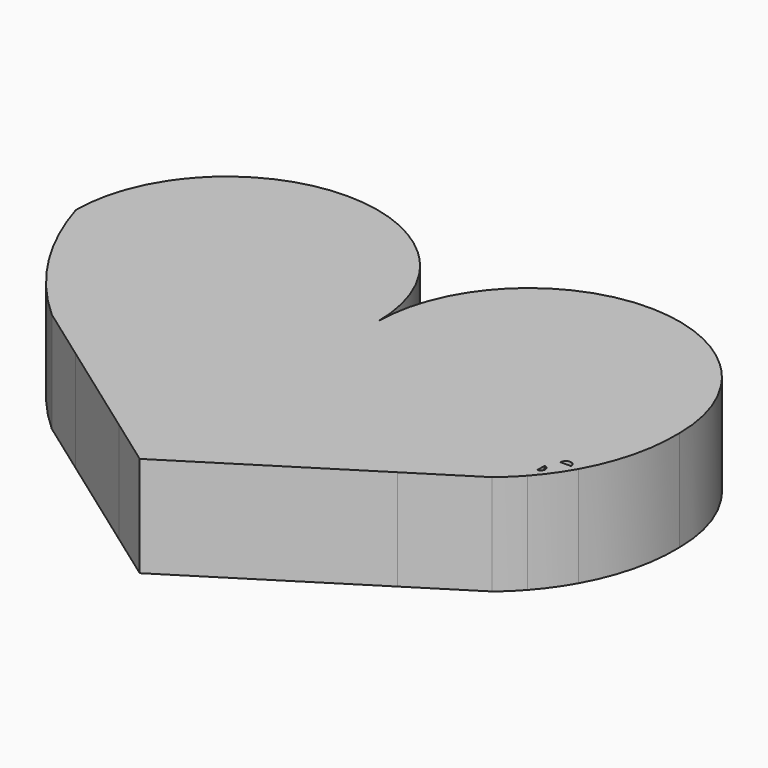
from build123d import *

# Parameters (mm, degrees)
F1_DEPTH = 25.4


with BuildPart() as f1:
    # F0 (on Top) → F1 (new body)
    with BuildSketch(Plane.XY):
        with BuildLine():
            Line((7.3731103912, 0), (0, 0))
            Line((0, 0), (-3.0946007464, 0))
            ThreePointArc((-3.0946007464, 0), (2.1392548224, -6.2743292812), (7.3731103912, 0))
        make_face()
        with BuildLine():
            ThreePointArc((69.9874537027, 20.8518655366), (67.2803767578, 24.4972572398), (64.1588523404, 27.7947155895))
            Line((64.1588523404, 27.7947155895), (64.1588523404, 25.8992332965))
            Line((64.1588523404, 25.8992332965), (64.1588523404, 20.8518655366))
            Line((64.1588523404, 20.8518655366), (65.8508837223, 20.8518655366))
            Line((65.8508837223, 20.8518655366), (68.7087923288, 20.8518655366))
            Line((68.7087923288, 20.8518655366), (69.9874537027, 20.8518655366))
        make_face()
        with BuildLine():
            ThreePointArc((13.9820705187, 29.494668629), (9.7658289741, 25.4712534493), (6.2125462973, 20.8518655366))
            Line((6.2125462973, 20.8518655366), (7.9780612141, 20.8518655366))
            ThreePointArc((7.9780612141, 20.8518655366), (10.7168983668, 23.5907026893), (13.4557355195, 20.8518655366))
            Line((13.4557355195, 20.8518655366), (13.9820705187, 20.8518655366))
            Line((13.9820705187, 20.8518655366), (13.9820705187, 23.8748770207))
            ThreePointArc((13.9820705187, 23.8748770207), (11.8386334758, 26.0183140635), (13.9820705187, 28.1617511064))
            Line((13.9820705187, 28.1617511064), (13.9820705187, 29.494668629))
        make_face()
        with BuildLine():
            Line((-8.6229192093, 20.8518655366), (-6.2125462973, 20.8518655366))
            ThreePointArc((-6.2125462973, 20.8518655366), (-9.0177469774, 24.613666105), (-12.2641128277, 28.0020880296))
            Line((-12.2641128277, 28.0020880296), (-12.2641128277, 25.3109112382))
            Line((-12.2641128277, 25.3109112382), (-12.2641128277, 22.7124486119))
            Line((-12.2641128277, 22.7124486119), (-12.2641128277, 20.8518655366))
            Line((-12.2641128277, 20.8518655366), (-10.6853200123, 20.8518655366))
            Line((-10.6853200123, 20.8518655366), (-8.6229192093, 20.8518655366))
        make_face()
        with BuildLine():
            Line((-64.0826212534, 25.3109112382), (-64.0826212534, 27.8659898945))
            ThreePointArc((-64.0826212534, 27.8659898945), (-67.2467987777, 24.5371987198), (-69.9874537027, 20.8518655366))
            Line((-69.9874537027, 20.8518655366), (-68.3164224029, 20.8518655366))
            ThreePointArc((-68.3164224029, 20.8518655366), (-66.9433735311, 22.1881347575), (-65.5703246593, 20.8518655366))
            Line((-65.5703246593, 20.8518655366), (-64.0826212534, 20.8518655366))
            Line((-64.0826212534, 20.8518655366), (-64.0826212534, 22.7124486119))
            ThreePointArc((-64.0826212534, 22.7124486119), (-65.3282893316, 24.011679925), (-64.0826212534, 25.3109112382))
        make_face()
        with BuildLine():
            Line((-72.4636018276, 0), (-76.2, 0))
            ThreePointArc((-76.2, 0), (-71.1383173271, -12.6890619161), (-64.0826212534, -24.3873556682))
            Line((-64.0826212534, -24.3873556682), (-64.0826212534, -17.1742849052))
            ThreePointArc((-64.0826212534, -17.1742849052), (-67.6059327944, -12.0701026171), (-64.0826212534, -6.9659203291))
            Line((-64.0826212534, -6.9659203291), (-64.0826212534, 0))
            Line((-64.0826212534, 0), (-66.7451322079, 0))
            ThreePointArc((-66.7451322079, 0), (-69.6043670177, -2.4147276963), (-72.4636018276, 0))
        make_face()
        with BuildLine():
            Line((-56.3778951764, -24.3873556682), (-64.0826212534, -24.3873556682))
            ThreePointArc((-64.0826212534, -24.3873556682), (-58.4160274717, -31.4204459437), (-52.0255934776, -37.8030000781))
            Line((-52.0255934776, -37.8030000781), (-38.1, -47.7827715515))
            Line((-38.1, -47.7827715515), (-38.1, -40.8103056252))
            ThreePointArc((-38.1, -40.8103056252), (-43.5800189721, -35.9057448804), (-38.1, -31.0011841357))
            Line((-38.1, -31.0011841357), (-38.1, -24.3873556682))
            Line((-38.1, -24.3873556682), (-45.1089218259, -24.3873556682))
            Line((-45.1089218259, -24.3873556682), (-56.3778951764, -24.3873556682))
        make_face()
        with BuildLine():
            ThreePointArc((64.1588523404, -32.9412611677), (67.4447841374, -28.8340923774), (70.2541819173, -24.3873556682))
            Line((70.2541819173, -24.3873556682), (68.3325305581, -24.3873556682))
            Line((68.3325305581, -24.3873556682), (65.6523033977, -24.3873556682))
            Line((65.6523033977, -24.3873556682), (64.1588523404, -24.3873556682))
            Line((64.1588523404, -24.3873556682), (64.1588523404, -27.585182339))
            ThreePointArc((64.1588523404, -27.585182339), (65.2624770419, -28.6888070405), (64.1588523404, -29.792431742))
            Line((64.1588523404, -29.792431742), (64.1588523404, -32.9412611677))
        make_face()
        with BuildLine():
            Line((-12.2641128277, -52.9070980847), (-12.2641128277, -47.7827715515))
            Line((-12.2641128277, -47.7827715515), (-18.7669228762, -47.7827715515))
            Line((-18.7669228762, -47.7827715515), (-29.9223959446, -47.7827715515))
            Line((-29.9223959446, -47.7827715515), (-38.1, -47.7827715515))
            Line((-38.1, -47.7827715515), (-12.2641128277, -66.2980506459))
            Line((-12.2641128277, -66.2980506459), (-12.2641128277, -61.5275651217))
            ThreePointArc((-12.2641128277, -61.5275651217), (-16.9211194514, -57.2173316032), (-12.2641128277, -52.9070980847))
        make_face()
        Polygon((21.1353525519, -47.7827715515), (13.9820705187, -47.7827715515), (13.9820705187, -54.9595914781), (13.9820705187, -60.7065707445), (13.9820705187, -66.2672672047), (43.2854445061, -47.7827715515), (35.3846773505, -47.7827715515), align=None)
        with BuildLine():
            ThreePointArc((76.2, 0), (74.6138465933, 10.878832978), (69.9874537027, 20.8518655366))
            Line((69.9874537027, 20.8518655366), (68.7087923288, 20.8518655366))
            ThreePointArc((68.7087923288, 20.8518655366), (67.2798380256, 19.4229112333), (65.8508837223, 20.8518655366))
            Line((65.8508837223, 20.8518655366), (64.1588523404, 20.8518655366))
            Line((64.1588523404, 20.8518655366), (64.1588523404, 15.7774444669))
            Line((64.1588523404, 15.7774444669), (64.1588523404, 4.3457765132))
            Line((64.1588523404, 4.3457765132), (64.1588523404, 0))
            Line((64.1588523404, 0), (76.2, 0))
        make_face()
        with BuildLine():
            ThreePointArc((70.2541819173, -24.3873556682), (74.8750675455, -12.5954667415), (76.2, 0))
            Line((76.2, 0), (64.1588523404, 0))
            Line((64.1588523404, 0), (64.1588523404, -7.877567783))
            ThreePointArc((64.1588523404, -7.877567783), (69.0336172821, -12.7523327246), (64.1588523404, -17.6270976663))
            Line((64.1588523404, -17.6270976663), (64.1588523404, -24.3873556682))
            Line((64.1588523404, -24.3873556682), (65.6523033977, -24.3873556682))
            ThreePointArc((65.6523033977, -24.3873556682), (66.9924169779, -23.0472420879), (68.3325305581, -24.3873556682))
            Line((68.3325305581, -24.3873556682), (70.2541819173, -24.3873556682))
        make_face()
        with BuildLine():
            ThreePointArc((64.1588523404, 27.7947155895), (54.4953024728, 34.3919184813), (43.2854445061, 37.7454787395))
            Line((43.2854445061, 37.7454787395), (43.2854445061, 33.5203446448))
            Line((43.2854445061, 33.5203446448), (43.2854445061, 24.9465927482))
            Line((43.2854445061, 24.9465927482), (43.2854445061, 20.8518655366))
            Line((43.2854445061, 20.8518655366), (48.5843010247, 20.8518655366))
            Line((48.5843010247, 20.8518655366), (60.2541230619, 20.8518655366))
            Line((60.2541230619, 20.8518655366), (63.1740450807, 20.8518655366))
            ThreePointArc((63.1740450807, 20.8518655366), (61.5875799588, 23.7811638152), (64.1588523404, 25.8992332965))
            Line((64.1588523404, 25.8992332965), (64.1588523404, 27.7947155895))
        make_face()
        with BuildLine():
            ThreePointArc((43.2854445061, 37.7454787395), (27.7738819635, 36.6739865067), (13.9820705187, 29.494668629))
            Line((13.9820705187, 29.494668629), (13.9820705187, 28.1617511064))
            Line((13.9820705187, 28.1617511064), (13.9820705187, 23.8748770207))
            Line((13.9820705187, 23.8748770207), (13.9820705187, 20.8518655366))
            Line((13.9820705187, 20.8518655366), (22.616366089, 20.8518655366))
            ThreePointArc((22.616366089, 20.8518655366), (28.9394616748, 27.1749611223), (35.2625572606, 20.8518655366))
            Line((35.2625572606, 20.8518655366), (43.2854445061, 20.8518655366))
            Line((43.2854445061, 20.8518655366), (43.2854445061, 24.9465927482))
            ThreePointArc((43.2854445061, 24.9465927482), (38.9985685578, 29.2334686965), (43.2854445061, 33.5203446448))
            Line((43.2854445061, 33.5203446448), (43.2854445061, 37.7454787395))
        make_face()
        with BuildLine():
            ThreePointArc((6.2125462973, 20.8518655366), (1.5861534067, 10.878832978), (0, 0))
            Line((0, 0), (7.3731103912, 0))
            Line((7.3731103912, 0), (13.9820705187, 0))
            Line((13.9820705187, 0), (13.9820705187, 4.531538114))
            Line((13.9820705187, 4.531538114), (13.9820705187, 13.5946199298))
            Line((13.9820705187, 13.5946199298), (13.9820705187, 20.8518655366))
            Line((13.9820705187, 20.8518655366), (13.4557355195, 20.8518655366))
            Line((13.4557355195, 20.8518655366), (7.9780612141, 20.8518655366))
            Line((7.9780612141, 20.8518655366), (6.2125462973, 20.8518655366))
        make_face()
        with BuildLine():
            Line((-3.0946007464, 0), (0, 0))
            ThreePointArc((0, 0), (-1.5861534067, 10.878832978), (-6.2125462973, 20.8518655366))
            Line((-6.2125462973, 20.8518655366), (-8.6229192093, 20.8518655366))
            ThreePointArc((-8.6229192093, 20.8518655366), (-9.6541196108, 18.7953565289), (-10.6853200123, 20.8518655366))
            Line((-10.6853200123, 20.8518655366), (-12.2641128277, 20.8518655366))
            Line((-12.2641128277, 20.8518655366), (-12.2641128277, 13.5718295351))
            ThreePointArc((-12.2641128277, 13.5718295351), (-6.9563915031, 10.103298584), (-12.2641128277, 6.6347676329))
            Line((-12.2641128277, 6.6347676329), (-12.2641128277, 0))
            Line((-12.2641128277, 0), (-3.0946007464, 0))
        make_face()
        with BuildLine():
            Line((-12.2641128277, 25.3109112382), (-12.2641128277, 28.0020880296))
            ThreePointArc((-12.2641128277, 28.0020880296), (-24.2304209496, 35.4858391047), (-38.1, 38.1))
            Line((-38.1, 38.1), (-38.1, 33.7021276355))
            Line((-38.1, 33.7021276355), (-38.1, 25.3109112382))
            Line((-38.1, 25.3109112382), (-38.1, 20.8518655366))
            Line((-38.1, 20.8518655366), (-32.246787101, 20.8518655366))
            Line((-32.246787101, 20.8518655366), (-17.6224876195, 20.8518655366))
            Line((-17.6224876195, 20.8518655366), (-12.2641128277, 20.8518655366))
            Line((-12.2641128277, 20.8518655366), (-12.2641128277, 22.7124486119))
            ThreePointArc((-12.2641128277, 22.7124486119), (-15.2984271998, 24.011679925), (-12.2641128277, 25.3109112382))
        make_face()
        with BuildLine():
            Line((-38.1, 33.7021276355), (-38.1, 38.1))
            ThreePointArc((-38.1, 38.1), (-52.0627322724, 35.4492892382), (-64.0826212534, 27.8659898945))
            Line((-64.0826212534, 27.8659898945), (-64.0826212534, 25.3109112382))
            Line((-64.0826212534, 25.3109112382), (-64.0826212534, 22.7124486119))
            Line((-64.0826212534, 22.7124486119), (-64.0826212534, 20.8518655366))
            Line((-64.0826212534, 20.8518655366), (-55.4025620222, 20.8518655366))
            ThreePointArc((-55.4025620222, 20.8518655366), (-49.9948691577, 25.7247809767), (-44.5871762931, 20.8518655366))
            Line((-44.5871762931, 20.8518655366), (-38.1, 20.8518655366))
            Line((-38.1, 20.8518655366), (-38.1, 25.3109112382))
            ThreePointArc((-38.1, 25.3109112382), (-43.0000966156, 29.5065194368), (-38.1, 33.7021276355))
        make_face()
        with BuildLine():
            Line((-68.3164224029, 20.8518655366), (-69.9874537027, 20.8518655366))
            ThreePointArc((-69.9874537027, 20.8518655366), (-74.6138465933, 10.878832978), (-76.2, 0))
            Line((-76.2, 0), (-72.4636018276, 0))
            Line((-72.4636018276, 0), (-66.7451322079, 0))
            Line((-66.7451322079, 0), (-64.0826212534, 0))
            Line((-64.0826212534, 0), (-64.0826212534, 5.2506080829))
            ThreePointArc((-64.0826212534, 5.2506080829), (-68.2045203392, 9.7503920551), (-64.0826212534, 14.2501760274))
            Line((-64.0826212534, 14.2501760274), (-64.0826212534, 20.8518655366))
            Line((-64.0826212534, 20.8518655366), (-65.5703246593, 20.8518655366))
            Line((-65.5703246593, 20.8518655366), (-68.3164224029, 20.8518655366))
        make_face()
        with BuildLine():
            Line((48.8840192556, -24.3873556682), (43.2854445061, -24.3873556682))
            Line((43.2854445061, -24.3873556682), (43.2854445061, -29.2515400797))
            Line((43.2854445061, -29.2515400797), (43.2854445061, -44.1332776099))
            Line((43.2854445061, -44.1332776099), (43.2854445061, -47.7827715515))
            Line((43.2854445061, -47.7827715515), (59.106323868, -37.8030000781))
            ThreePointArc((59.106323868, -37.8030000781), (61.7228361509, -35.46592028), (64.1588523404, -32.9412611677))
            Line((64.1588523404, -32.9412611677), (64.1588523404, -29.792431742))
            Line((64.1588523404, -29.792431742), (64.1588523404, -27.585182339))
            Line((64.1588523404, -27.585182339), (64.1588523404, -24.3873556682))
            Line((64.1588523404, -24.3873556682), (63.8832971454, -24.3873556682))
            ThreePointArc((63.8832971454, -24.3873556682), (56.3836582005, -31.886994613), (48.8840192556, -24.3873556682))
        make_face()
        with BuildLine():
            Line((13.9820705187, -54.9595914781), (13.9820705187, -47.7827715515))
            Line((13.9820705187, -47.7827715515), (5.5258679204, -47.7827715515))
            ThreePointArc((5.5258679204, -47.7827715515), (-0.3237351775, -55.877302251), (-6.1733382754, -47.7827715515))
            Line((-6.1733382754, -47.7827715515), (-12.2641128277, -47.7827715515))
            Line((-12.2641128277, -47.7827715515), (-12.2641128277, -52.9070980847))
            Line((-12.2641128277, -52.9070980847), (-12.2641128277, -61.5275651217))
            Line((-12.2641128277, -61.5275651217), (-12.2641128277, -66.2980506459))
            Line((-12.2641128277, -66.2980506459), (0, -75.0871226192))
            Line((0, -75.0871226192), (13.9820705187, -66.2672672047))
            Line((13.9820705187, -66.2672672047), (13.9820705187, -60.7065707445))
            ThreePointArc((13.9820705187, -60.7065707445), (8.35846738, -57.8330811113), (13.9820705187, -54.9595914781))
        make_face()
        with BuildLine():
            Line((-38.1, -6.2933946028), (-38.1, 0))
            Line((-38.1, 0), (-46.1211204529, 0))
            Line((-46.1211204529, 0), (-55.3081780672, 0))
            Line((-55.3081780672, 0), (-64.0826212534, 0))
            Line((-64.0826212534, 0), (-64.0826212534, -6.9659203291))
            Line((-64.0826212534, -6.9659203291), (-64.0826212534, -17.1742849052))
            Line((-64.0826212534, -17.1742849052), (-64.0826212534, -24.3873556682))
            Line((-64.0826212534, -24.3873556682), (-56.3778951764, -24.3873556682))
            ThreePointArc((-56.3778951764, -24.3873556682), (-50.7434085011, -16.8907498785), (-45.1089218259, -24.3873556682))
            Line((-45.1089218259, -24.3873556682), (-38.1, -24.3873556682))
            Line((-38.1, -24.3873556682), (-38.1, -20.0098585337))
            Line((-38.1, -20.0098585337), (-38.1, -6.2933946028))
        make_face()
        with BuildLine():
            Line((-12.2641128277, -32.1551971138), (-12.2641128277, -24.3873556682))
            Line((-12.2641128277, -24.3873556682), (-20.3056093305, -24.3873556682))
            ThreePointArc((-20.3056093305, -24.3873556682), (-24.0561561659, -29.287069319), (-27.8067030013, -24.3873556682))
            Line((-27.8067030013, -24.3873556682), (-38.1, -24.3873556682))
            Line((-38.1, -24.3873556682), (-38.1, -31.0011841357))
            Line((-38.1, -31.0011841357), (-38.1, -40.8103056252))
            Line((-38.1, -40.8103056252), (-38.1, -47.7827715515))
            Line((-38.1, -47.7827715515), (-29.9223959446, -47.7827715515))
            ThreePointArc((-29.9223959446, -47.7827715515), (-24.3446594104, -38.7493341849), (-18.7669228762, -47.7827715515))
            Line((-18.7669228762, -47.7827715515), (-12.2641128277, -47.7827715515))
            Line((-12.2641128277, -47.7827715515), (-12.2641128277, -41.0026423633))
            Line((-12.2641128277, -41.0026423633), (-12.2641128277, -32.1551971138))
        make_face()
        with BuildLine():
            Line((21.5103328228, -24.3873556682), (13.9820705187, -24.3873556682))
            Line((13.9820705187, -24.3873556682), (13.9820705187, -31.7664258182))
            Line((13.9820705187, -31.7664258182), (13.9820705187, -41.6183918715))
            Line((13.9820705187, -41.6183918715), (13.9820705187, -47.7827715515))
            Line((13.9820705187, -47.7827715515), (21.1353525519, -47.7827715515))
            ThreePointArc((21.1353525519, -47.7827715515), (28.2600149512, -40.6581091522), (35.3846773505, -47.7827715515))
            Line((35.3846773505, -47.7827715515), (43.2854445061, -47.7827715515))
            Line((43.2854445061, -47.7827715515), (43.2854445061, -44.1332776099))
            ThreePointArc((43.2854445061, -44.1332776099), (35.844575741, -36.6924088448), (43.2854445061, -29.2515400797))
            Line((43.2854445061, -29.2515400797), (43.2854445061, -24.3873556682))
            Line((43.2854445061, -24.3873556682), (35.7596613467, -24.3873556682))
            Line((35.7596613467, -24.3873556682), (21.5103328228, -24.3873556682))
        make_face()
        with BuildLine():
            Line((13.9820705187, 0), (7.3731103912, 0))
            ThreePointArc((7.3731103912, 0), (2.1392548224, -6.2743292812), (-3.0946007464, 0))
            Line((-3.0946007464, 0), (-12.2641128277, 0))
            Line((-12.2641128277, 0), (-12.2641128277, -8.9736226946))
            ThreePointArc((-12.2641128277, -8.9736226946), (-8.4361824744, -13.0727961659), (-12.2641128277, -17.1719696373))
            Line((-12.2641128277, -17.1719696373), (-12.2641128277, -24.3873556682))
            Line((-12.2641128277, -24.3873556682), (-7.1995845065, -24.3873556682))
            Line((-7.1995845065, -24.3873556682), (6.9626118056, -24.3873556682))
            Line((6.9626118056, -24.3873556682), (13.9820705187, -24.3873556682))
            Line((13.9820705187, -24.3873556682), (13.9820705187, -18.3862992879))
            Line((13.9820705187, -18.3862992879), (13.9820705187, -9.394259192))
            Line((13.9820705187, -9.394259192), (13.9820705187, 0))
        make_face()
        with BuildLine():
            Line((-12.2641128277, -8.9736226946), (-12.2641128277, 0))
            Line((-12.2641128277, 0), (-19.0984625369, 0))
            ThreePointArc((-19.0984625369, 0), (-24.9319020659, -6.3078507166), (-30.7653415948, 0))
            Line((-30.7653415948, 0), (-38.1, 0))
            Line((-38.1, 0), (-38.1, -6.2933946028))
            ThreePointArc((-38.1, -6.2933946028), (-32.493432726, -13.1516265683), (-38.1, -20.0098585337))
            Line((-38.1, -20.0098585337), (-38.1, -24.3873556682))
            Line((-38.1, -24.3873556682), (-27.8067030013, -24.3873556682))
            Line((-27.8067030013, -24.3873556682), (-20.3056093305, -24.3873556682))
            Line((-20.3056093305, -24.3873556682), (-12.2641128277, -24.3873556682))
            Line((-12.2641128277, -24.3873556682), (-12.2641128277, -17.1719696373))
            Line((-12.2641128277, -17.1719696373), (-12.2641128277, -8.9736226946))
        make_face()
        with BuildLine():
            Line((20.543390885, 0), (13.9820705187, 0))
            Line((13.9820705187, 0), (13.9820705187, -9.394259192))
            ThreePointArc((13.9820705187, -9.394259192), (20.7282060591, -13.89027924), (13.9820705187, -18.3862992879))
            Line((13.9820705187, -18.3862992879), (13.9820705187, -24.3873556682))
            Line((13.9820705187, -24.3873556682), (21.5103328228, -24.3873556682))
            ThreePointArc((21.5103328228, -24.3873556682), (28.6349970847, -17.2626914062), (35.7596613467, -24.3873556682))
            Line((35.7596613467, -24.3873556682), (43.2854445061, -24.3873556682))
            Line((43.2854445061, -24.3873556682), (43.2854445061, -21.2359833103))
            ThreePointArc((43.2854445061, -21.2359833103), (35.176776054, -13.1273148581), (43.2854445061, -5.018646406))
            Line((43.2854445061, -5.018646406), (43.2854445061, 0))
            Line((43.2854445061, 0), (31.3057955354, 0))
            Line((31.3057955354, 0), (20.543390885, 0))
        make_face()
        Polygon((47.1553392708, 0), (43.2854445061, 0), (43.2854445061, -5.018646406), (43.2854445061, -21.2359833103), (43.2854445061, -24.3873556682), (48.8840192556, -24.3873556682), (63.8832971454, -24.3873556682), (64.1588523404, -24.3873556682), (64.1588523404, -17.6270976663), (64.1588523404, -7.877567783), (64.1588523404, 0), (60.4922883213, 0), align=None)
        with BuildLine():
            Line((13.9820705187, 4.531538114), (13.9820705187, 0))
            Line((13.9820705187, 0), (20.543390885, 0))
            ThreePointArc((20.543390885, 0), (25.9245932102, 5.3812023252), (31.3057955354, 0))
            Line((31.3057955354, 0), (43.2854445061, 0))
            Line((43.2854445061, 0), (43.2854445061, 9.0630790219))
            ThreePointArc((43.2854445061, 9.0630790219), (38.119115994, 14.229407534), (43.2854445061, 19.3957360461))
            Line((43.2854445061, 19.3957360461), (43.2854445061, 20.8518655366))
            Line((43.2854445061, 20.8518655366), (35.2625572606, 20.8518655366))
            Line((35.2625572606, 20.8518655366), (22.616366089, 20.8518655366))
            Line((22.616366089, 20.8518655366), (13.9820705187, 20.8518655366))
            Line((13.9820705187, 20.8518655366), (13.9820705187, 13.5946199298))
            ThreePointArc((13.9820705187, 13.5946199298), (18.5136114266, 9.0630790219), (13.9820705187, 4.531538114))
        make_face()
        with BuildLine():
            Line((43.2854445061, 9.0630790219), (43.2854445061, 0))
            Line((43.2854445061, 0), (47.1553392708, 0))
            ThreePointArc((47.1553392708, 0), (53.823813796, 6.6684745252), (60.4922883213, 0))
            Line((60.4922883213, 0), (64.1588523404, 0))
            Line((64.1588523404, 0), (64.1588523404, 4.3457765132))
            ThreePointArc((64.1588523404, 4.3457765132), (58.4430183636, 10.0616104901), (64.1588523404, 15.7774444669))
            Line((64.1588523404, 15.7774444669), (64.1588523404, 20.8518655366))
            Line((64.1588523404, 20.8518655366), (63.1740450807, 20.8518655366))
            Line((63.1740450807, 20.8518655366), (60.2541230619, 20.8518655366))
            ThreePointArc((60.2541230619, 20.8518655366), (54.4192120433, 15.016954518), (48.5843010247, 20.8518655366))
            Line((48.5843010247, 20.8518655366), (43.2854445061, 20.8518655366))
            Line((43.2854445061, 20.8518655366), (43.2854445061, 19.3957360461))
            Line((43.2854445061, 19.3957360461), (43.2854445061, 9.0630790219))
        make_face()
        with BuildLine():
            Line((-19.0984625369, 0), (-12.2641128277, 0))
            Line((-12.2641128277, 0), (-12.2641128277, 6.6347676329))
            Line((-12.2641128277, 6.6347676329), (-12.2641128277, 13.5718295351))
            Line((-12.2641128277, 13.5718295351), (-12.2641128277, 20.8518655366))
            Line((-12.2641128277, 20.8518655366), (-17.6224876195, 20.8518655366))
            ThreePointArc((-17.6224876195, 20.8518655366), (-24.9346373603, 15.1396827417), (-32.246787101, 20.8518655366))
            Line((-32.246787101, 20.8518655366), (-38.1, 20.8518655366))
            Line((-38.1, 20.8518655366), (-38.1, 14.0626849607))
            ThreePointArc((-38.1, 14.0626849607), (-33.6929838401, 9.2347918544), (-38.1, 4.4068987481))
            Line((-38.1, 4.4068987481), (-38.1, 0))
            Line((-38.1, 0), (-30.7653415948, 0))
            Line((-30.7653415948, 0), (-19.0984625369, 0))
        make_face()
        with BuildLine():
            Line((-46.1211204529, 0), (-38.1, 0))
            Line((-38.1, 0), (-38.1, 4.4068987481))
            Line((-38.1, 4.4068987481), (-38.1, 14.0626849607))
            Line((-38.1, 14.0626849607), (-38.1, 20.8518655366))
            Line((-38.1, 20.8518655366), (-44.5871762931, 20.8518655366))
            Line((-44.5871762931, 20.8518655366), (-55.4025620222, 20.8518655366))
            Line((-55.4025620222, 20.8518655366), (-64.0826212534, 20.8518655366))
            Line((-64.0826212534, 20.8518655366), (-64.0826212534, 14.2501760274))
            Line((-64.0826212534, 14.2501760274), (-64.0826212534, 5.2506080829))
            Line((-64.0826212534, 5.2506080829), (-64.0826212534, 0))
            Line((-64.0826212534, 0), (-55.3081780672, 0))
            ThreePointArc((-55.3081780672, 0), (-50.71464926, 4.1266133924), (-46.1211204529, 0))
        make_face()
        with BuildLine():
            Line((13.9820705187, -31.7664258182), (13.9820705187, -24.3873556682))
            Line((13.9820705187, -24.3873556682), (6.9626118056, -24.3873556682))
            ThreePointArc((6.9626118056, -24.3873556682), (-0.1184863504, -31.8409854663), (-7.1995845065, -24.3873556682))
            Line((-7.1995845065, -24.3873556682), (-12.2641128277, -24.3873556682))
            Line((-12.2641128277, -24.3873556682), (-12.2641128277, -32.1551971138))
            ThreePointArc((-12.2641128277, -32.1551971138), (-6.9831720335, -36.5789197385), (-12.2641128277, -41.0026423633))
            Line((-12.2641128277, -41.0026423633), (-12.2641128277, -47.7827715515))
            Line((-12.2641128277, -47.7827715515), (-6.1733382754, -47.7827715515))
            Line((-6.1733382754, -47.7827715515), (5.5258679204, -47.7827715515))
            Line((5.5258679204, -47.7827715515), (13.9820705187, -47.7827715515))
            Line((13.9820705187, -47.7827715515), (13.9820705187, -41.6183918715))
            ThreePointArc((13.9820705187, -41.6183918715), (4.354912737, -36.6924088448), (13.9820705187, -31.7664258182))
        make_face()
        with BuildLine():
            ThreePointArc((-10.6853200123, 20.8518655366), (-9.6541196108, 18.7953565289), (-8.6229192093, 20.8518655366))
            Line((-8.6229192093, 20.8518655366), (-10.6853200123, 20.8518655366))
        make_face()
        with BuildLine():
            Line((-12.2641128277, 22.7124486119), (-12.2641128277, 25.3109112382))
            ThreePointArc((-12.2641128277, 25.3109112382), (-15.2984271998, 24.011679925), (-12.2641128277, 22.7124486119))
        make_face()
        with BuildLine():
            ThreePointArc((-32.246787101, 20.8518655366), (-24.9346373603, 15.1396827417), (-17.6224876195, 20.8518655366))
            Line((-17.6224876195, 20.8518655366), (-32.246787101, 20.8518655366))
        make_face()
        with BuildLine():
            Line((-12.2641128277, 13.5718295351), (-12.2641128277, 6.6347676329))
            ThreePointArc((-12.2641128277, 6.6347676329), (-6.9563915031, 10.103298584), (-12.2641128277, 13.5718295351))
        make_face()
        with BuildLine():
            ThreePointArc((-30.7653415948, 0), (-24.9319020659, -6.3078507166), (-19.0984625369, 0))
            Line((-19.0984625369, 0), (-30.7653415948, 0))
        make_face()
        with BuildLine():
            Line((-38.1, 14.0626849607), (-38.1, 4.4068987481))
            ThreePointArc((-38.1, 4.4068987481), (-33.6929838401, 9.2347918544), (-38.1, 14.0626849607))
        make_face()
        with BuildLine():
            Line((-38.1, 25.3109112382), (-38.1, 33.7021276355))
            ThreePointArc((-38.1, 33.7021276355), (-43.0000966156, 29.5065194368), (-38.1, 25.3109112382))
        make_face()
        with BuildLine():
            Line((-55.4025620222, 20.8518655366), (-44.5871762931, 20.8518655366))
            ThreePointArc((-44.5871762931, 20.8518655366), (-49.9948691577, 25.7247809767), (-55.4025620222, 20.8518655366))
        make_face()
        with BuildLine():
            Line((-64.0826212534, 22.7124486119), (-64.0826212534, 25.3109112382))
            ThreePointArc((-64.0826212534, 25.3109112382), (-65.3282893316, 24.011679925), (-64.0826212534, 22.7124486119))
        make_face()
        with BuildLine():
            ThreePointArc((-65.5703246593, 20.8518655366), (-66.9433735311, 22.1881347575), (-68.3164224029, 20.8518655366))
            Line((-68.3164224029, 20.8518655366), (-65.5703246593, 20.8518655366))
        make_face()
        with BuildLine():
            Line((-64.0826212534, 5.2506080829), (-64.0826212534, 14.2501760274))
            ThreePointArc((-64.0826212534, 14.2501760274), (-68.2045203392, 9.7503920551), (-64.0826212534, 5.2506080829))
        make_face()
        with BuildLine():
            Line((-66.7451322079, 0), (-72.4636018276, 0))
            ThreePointArc((-72.4636018276, 0), (-69.6043670177, -2.4147276963), (-66.7451322079, 0))
        make_face()
        with BuildLine():
            ThreePointArc((-64.0826212534, -6.9659203291), (-67.6059327944, -12.0701026171), (-64.0826212534, -17.1742849052))
            Line((-64.0826212534, -17.1742849052), (-64.0826212534, -6.9659203291))
        make_face()
        with BuildLine():
            ThreePointArc((-45.1089218259, -24.3873556682), (-50.7434085011, -16.8907498785), (-56.3778951764, -24.3873556682))
            Line((-56.3778951764, -24.3873556682), (-45.1089218259, -24.3873556682))
        make_face()
        with BuildLine():
            ThreePointArc((-38.1, -20.0098585337), (-32.493432726, -13.1516265683), (-38.1, -6.2933946028))
            Line((-38.1, -6.2933946028), (-38.1, -20.0098585337))
        make_face()
        with BuildLine():
            Line((-55.3081780672, 0), (-46.1211204529, 0))
            ThreePointArc((-46.1211204529, 0), (-50.71464926, 4.1266133924), (-55.3081780672, 0))
        make_face()
        with BuildLine():
            ThreePointArc((-12.2641128277, -17.1719696373), (-8.4361824744, -13.0727961659), (-12.2641128277, -8.9736226946))
            Line((-12.2641128277, -8.9736226946), (-12.2641128277, -17.1719696373))
        make_face()
        with BuildLine():
            ThreePointArc((-27.8067030013, -24.3873556682), (-24.0561561659, -29.287069319), (-20.3056093305, -24.3873556682))
            Line((-20.3056093305, -24.3873556682), (-27.8067030013, -24.3873556682))
        make_face()
        with BuildLine():
            Line((-38.1, -40.8103056252), (-38.1, -31.0011841357))
            ThreePointArc((-38.1, -31.0011841357), (-43.5800189721, -35.9057448804), (-38.1, -40.8103056252))
        make_face()
        with BuildLine():
            Line((-29.9223959446, -47.7827715515), (-18.7669228762, -47.7827715515))
            ThreePointArc((-18.7669228762, -47.7827715515), (-24.3446594104, -38.7493341849), (-29.9223959446, -47.7827715515))
        make_face()
        with BuildLine():
            ThreePointArc((-12.2641128277, -41.0026423633), (-6.9831720335, -36.5789197385), (-12.2641128277, -32.1551971138))
            Line((-12.2641128277, -32.1551971138), (-12.2641128277, -41.0026423633))
        make_face()
        with BuildLine():
            ThreePointArc((-7.1995845065, -24.3873556682), (-0.1184863504, -31.8409854663), (6.9626118056, -24.3873556682))
            Line((6.9626118056, -24.3873556682), (-7.1995845065, -24.3873556682))
        make_face()
        with BuildLine():
            Line((13.9820705187, -41.6183918715), (13.9820705187, -31.7664258182))
            ThreePointArc((13.9820705187, -31.7664258182), (4.354912737, -36.6924088448), (13.9820705187, -41.6183918715))
        make_face()
        with BuildLine():
            ThreePointArc((-6.1733382754, -47.7827715515), (-0.3237351775, -55.877302251), (5.5258679204, -47.7827715515))
            Line((5.5258679204, -47.7827715515), (-6.1733382754, -47.7827715515))
        make_face()
        with BuildLine():
            Line((13.9820705187, -60.7065707445), (13.9820705187, -54.9595914781))
            ThreePointArc((13.9820705187, -54.9595914781), (8.35846738, -57.8330811113), (13.9820705187, -60.7065707445))
        make_face()
        with BuildLine():
            Line((-12.2641128277, -61.5275651217), (-12.2641128277, -52.9070980847))
            ThreePointArc((-12.2641128277, -52.9070980847), (-16.9211194514, -57.2173316032), (-12.2641128277, -61.5275651217))
        make_face()
        with BuildLine():
            ThreePointArc((35.3846773505, -47.7827715515), (28.2600149512, -40.6581091522), (21.1353525519, -47.7827715515))
            Line((21.1353525519, -47.7827715515), (35.3846773505, -47.7827715515))
        make_face()
        with BuildLine():
            Line((43.2854445061, -44.1332776099), (43.2854445061, -29.2515400797))
            ThreePointArc((43.2854445061, -29.2515400797), (35.844575741, -36.6924088448), (43.2854445061, -44.1332776099))
        make_face()
        with BuildLine():
            ThreePointArc((35.7596613467, -24.3873556682), (28.6349970847, -17.2626914062), (21.5103328228, -24.3873556682))
            Line((21.5103328228, -24.3873556682), (35.7596613467, -24.3873556682))
        make_face()
        with BuildLine():
            ThreePointArc((64.1588523404, -17.6270976663), (69.0336172821, -12.7523327246), (64.1588523404, -7.877567783))
            Line((64.1588523404, -7.877567783), (64.1588523404, -17.6270976663))
        make_face()
        with BuildLine():
            Line((43.2854445061, -21.2359833103), (43.2854445061, -5.018646406))
            ThreePointArc((43.2854445061, -5.018646406), (35.176776054, -13.1273148581), (43.2854445061, -21.2359833103))
        make_face()
        with BuildLine():
            ThreePointArc((31.3057955354, 0), (25.9245932102, 5.3812023252), (20.543390885, 0))
            Line((20.543390885, 0), (31.3057955354, 0))
        make_face()
        with BuildLine():
            Line((13.9820705187, 13.5946199298), (13.9820705187, 4.531538114))
            ThreePointArc((13.9820705187, 4.531538114), (18.5136114266, 9.0630790219), (13.9820705187, 13.5946199298))
        make_face()
        with BuildLine():
            ThreePointArc((43.2854445061, 19.3957360461), (38.119115994, 14.229407534), (43.2854445061, 9.0630790219))
            Line((43.2854445061, 9.0630790219), (43.2854445061, 19.3957360461))
        make_face()
        with BuildLine():
            ThreePointArc((48.5843010247, 20.8518655366), (54.4192120433, 15.016954518), (60.2541230619, 20.8518655366))
            Line((60.2541230619, 20.8518655366), (48.5843010247, 20.8518655366))
        make_face()
        with BuildLine():
            Line((64.1588523404, 4.3457765132), (64.1588523404, 15.7774444669))
            ThreePointArc((64.1588523404, 15.7774444669), (58.4430183636, 10.0616104901), (64.1588523404, 4.3457765132))
        make_face()
        with BuildLine():
            ThreePointArc((60.4922883213, 0), (53.823813796, 6.6684745252), (47.1553392708, 0))
            Line((47.1553392708, 0), (60.4922883213, 0))
        make_face()
        with BuildLine():
            ThreePointArc((13.9820705187, -18.3862992879), (20.7282060591, -13.89027924), (13.9820705187, -9.394259192))
            Line((13.9820705187, -9.394259192), (13.9820705187, -18.3862992879))
        make_face()
        with BuildLine():
            Line((64.1588523404, 20.8518655366), (64.1588523404, 25.8992332965))
            ThreePointArc((64.1588523404, 25.8992332965), (61.5875799588, 23.7811638152), (63.1740450807, 20.8518655366))
            Line((63.1740450807, 20.8518655366), (64.1588523404, 20.8518655366))
        make_face()
        with BuildLine():
            ThreePointArc((65.8508837223, 20.8518655366), (67.2798380256, 19.4229112333), (68.7087923288, 20.8518655366))
            Line((68.7087923288, 20.8518655366), (65.8508837223, 20.8518655366))
        make_face()
        with BuildLine():
            ThreePointArc((35.2625572606, 20.8518655366), (28.9394616748, 27.1749611223), (22.616366089, 20.8518655366))
            Line((22.616366089, 20.8518655366), (35.2625572606, 20.8518655366))
        make_face()
        with BuildLine():
            Line((13.9820705187, 23.8748770207), (13.9820705187, 28.1617511064))
            ThreePointArc((13.9820705187, 28.1617511064), (11.8386334758, 26.0183140635), (13.9820705187, 23.8748770207))
        make_face()
        with BuildLine():
            ThreePointArc((13.4557355195, 20.8518655366), (10.7168983668, 23.5907026893), (7.9780612141, 20.8518655366))
            Line((7.9780612141, 20.8518655366), (13.4557355195, 20.8518655366))
        make_face()
        with BuildLine():
            Line((43.2854445061, 24.9465927482), (43.2854445061, 33.5203446448))
            ThreePointArc((43.2854445061, 33.5203446448), (38.9985685578, 29.2334686965), (43.2854445061, 24.9465927482))
        make_face()
        with BuildLine():
            Line((63.8832971454, -24.3873556682), (48.8840192556, -24.3873556682))
            ThreePointArc((48.8840192556, -24.3873556682), (56.3836582005, -31.886994613), (63.8832971454, -24.3873556682))
        make_face()
    extrude(amount=F1_DEPTH)


solid = f1.part
